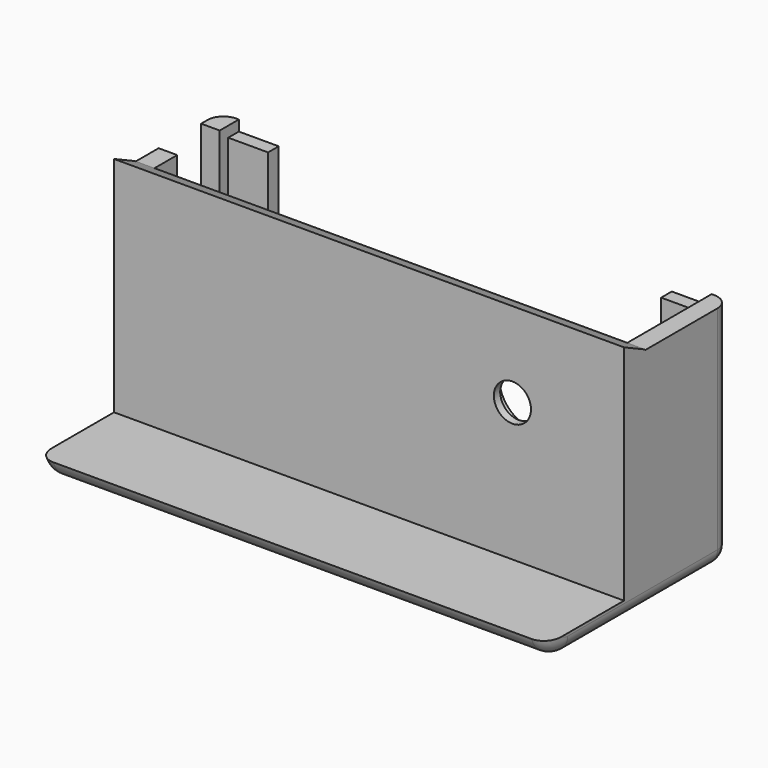
from build123d import *

# Parameters (mm, degrees)
F0_W           = 96
F0_H           = 43
F1_DEPTH       = 3.5
F2_T1_DEPTH    = 119.8484800354
F4_DEPTH       = 42
F5_T1_DEPTH    = 122.0704317696
F7_D           = 7
F7_CBORE_D     = 13
F7_CBORE_DEPTH = 3.5
F8_DEPTH       = 39.5
F3_W           = 89
F3_H           = 2.5
F9_DEPTH       = 3
F10_W          = 7.5
F10_H          = 2.5
F11_DEPTH      = 34.5
F12_W          = 10
F12_H          = 35
F13_DEPTH      = 3.5
F14_R          = 3


# Not quite as in the source:
# - a fillet or chamfer that OpenCascade refuses, or shapes differently, is made with other operations: its cross-section is extruded or revolved along the edge and cut away or added


with BuildPart() as f1:
    # F0 (on Top) → F1 (new body)
    with BuildSketch(Plane.XY):
        Rectangle(F0_W, F0_H)
    extrude(amount=F1_DEPTH)

    # F2: fillet of radius 5 on 1 edges, made by hand

    # F2_s2 → F2_t1 (cut)
    with BuildSketch(Plane.YZ.offset(-59.9242400177)):
        with BuildLine():
            ThreePointArc((-21.5, 3.5), (-19.6883438845, 0.9688711259), (-16.7303039929, 0))
            Line((-16.7303039929, 0), (-21.5, 0))
            Line((-21.5, 0), (-21.5, 3.5))
        make_face()
    extrude(amount=F2_T1_DEPTH, mode=Mode.SUBTRACT)

    # F3 (on face) → F4 (join)
    with BuildSketch(Plane.XY.offset(3.5)):
        Polygon((-48, 1.5), (-48, -3.5), (48, -3.5), (48, 1.5), (44.5, 1.5), (-44.5, 1.5), align=None)
    extrude(amount=F4_DEPTH)

    # F5: chamfer of 2.4 x 5.0317046378 on 1 edges, made by hand

    # F5_s2 → F5_t1 (cut)
    with BuildSketch(Plane.YZ.offset(-61.0352158848)):
        Polygon((1.5, 43.1), (-3.5317046378, 45.5), (1.5, 45.5), align=None)
    extrude(amount=F5_T1_DEPTH, mode=Mode.SUBTRACT)

    # F7 (through all)
    with Locations(Plane(origin=(0, 1.5, 0), x_dir=(-1, 0, 0), z_dir=(0, 1, 0))):
        with Locations((-27, 29.5)):
            CounterBoreHole(F7_D / 2, F7_CBORE_D / 2, F7_CBORE_DEPTH)

    # F3 (on face) → F8 (join)
    with BuildSketch(Plane.XY.offset(3.5)):
        Polygon((44.5, 1.5), (48, 1.5), (48, 21.5), (44.5, 21.5), (44.5, 19), align=None)
        Polygon((-48, 21.5), (-48, 1.5), (-44.5, 1.5), (-44.5, 19), (-44.5, 21.5), align=None)
    extrude(amount=F8_DEPTH)

    # F3 (on face) → F9 (join)
    with BuildSketch(Plane.XY.offset(3.5)):
        with Locations((0, 20.25)):
            Rectangle(F3_W, F3_H)
    extrude(amount=F9_DEPTH)

    # F10 (on face) → F11 (join)
    with BuildSketch(Plane.XY.offset(6.5)):
        with Locations((40.75, 20.25)):
            Rectangle(F10_W, F10_H)
        with Locations((-40.75, 20.25)):
            Rectangle(F10_W, F10_H)
    extrude(amount=F11_DEPTH)

    # F12 (on face) → F13 (cut)
    with BuildSketch(Plane.YZ.offset(-44.5)):
        with Locations((12, 25.5)):
            Rectangle(F12_W, F12_H)
    extrude(amount=-F13_DEPTH, mode=Mode.SUBTRACT)

    # F14
    f14_edges = [f1.edges().sort_by_distance(p)[0] for p in [
        (-48, 21.5, 21.5),
        (48, 21.5, 21.5),
        (-48, -19.688344, 0.968871),
        (48, -19.688344, 0.968871),
        (0, 21.5, 0),
        (48, 2.384848, 0),
        (-48, 2.384848, 0),
    ]]
    fillet(f14_edges, radius=F14_R)


solid = f1.part
